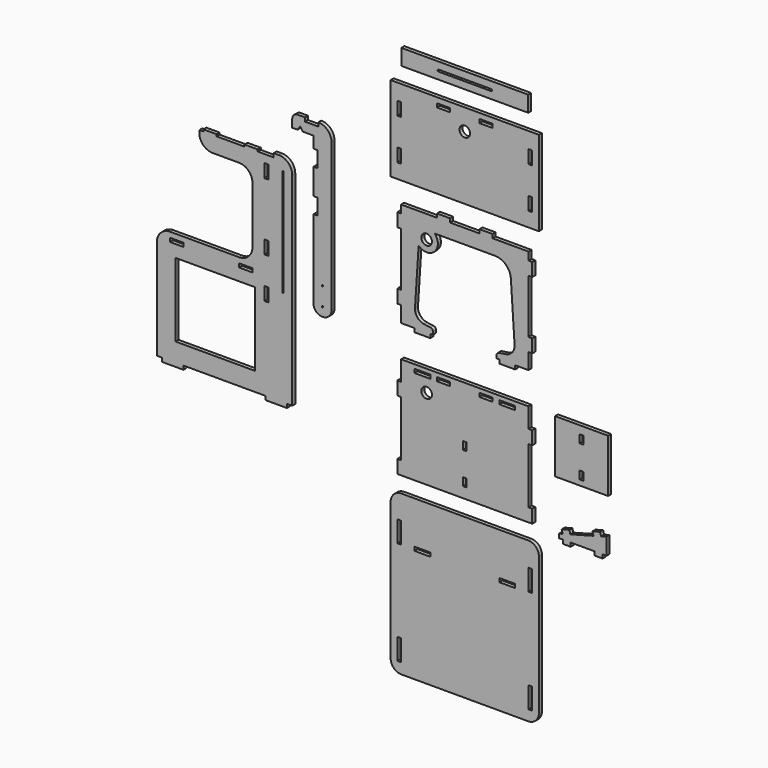
from build123d import *

# Parameters (mm, degrees)
F1_W     = 381
F1_H     = 352.425
F1_W_2   = 63.5
F1_H_2   = 18.034
F1_W_3   = 18.034
F1_H_3   = 63.5
F1_H_4   = 9.017
F1_W_4   = 101.6
F2_DEPTH = 18.034
F1_W_5   = 76.2
F1_H_5   = 38.1
F1_R     = 25.4
F1_H_6   = 101.6
F1_W_6   = 709.168
F1_H_7   = 406.4
F1_R_2   = 3.302
F1_W_7   = 607.06
F1_H_8   = 76.2
F1_W_8   = 254
F1_H_9   = 254
F1_W_9   = 38.1


# Not quite as in the source:
# - a variable given as a bare number and used for a length is read in inches; the dataset says mm whatever the document's units were
# - a feature names something its author has since deleted; it is built from what else it names


with BuildPart() as f2:
    # F1 (on Front) → F2 (new body)
    with BuildSketch(Plane.XZ):
        with BuildLine():
            Line((-279.4, -155.575), (-279.4, -635))
            Line((-279.4, -635), (-254, -635))
            Line((-254, -635), (-152.4, -635))
            Line((-152.4, -635), (241.3, -635))
            Line((241.3, -635), (279.4, -635))
            Line((279.4, -635), (342.9, -635))
            Line((342.9, -635), (368.3, -635))
            Line((368.3, -635), (368.3, 336.55))
            ThreePointArc((368.3, 336.55), (349.7012806053, 381.4512806053), (304.8, 400.05))
            Line((304.8, 400.05), (279.4, 400.05))
            Line((279.4, 400.05), (279.4, 382.016))
            Line((279.4, 382.016), (203.2, 382.016))
            Line((203.2, 382.016), (139.7, 382.016))
            Line((139.7, 382.016), (6.35, 382.016))
            Line((6.35, 382.016), (-57.15, 382.016))
            Line((-57.15, 382.016), (-76.2, 382.016))
            Line((-76.2, 382.016), (-76.2, 369.316))
            ThreePointArc((-76.2, 369.316), (-57.6012806053, 324.4147193947), (-12.7, 305.816))
            Line((-12.7, 305.816), (114.3, 305.816))
            ThreePointArc((114.3, 305.816), (159.2012806053, 287.2172806053), (177.8, 242.316))
            Line((177.8, 242.316), (177.8, -28.575))
            ThreePointArc((177.8, -28.575), (159.2012806053, -73.4762806053), (114.3, -92.075))
            Line((114.3, -92.075), (-215.9, -92.075))
            ThreePointArc((-215.9, -92.075), (-260.8012806053, -110.6737193947), (-279.4, -155.575))
        make_face()
        with Locations((0, -369.8875)):
            Rectangle(F1_W, F1_H, mode=Mode.SUBTRACT)
        with Locations((-184.15, -126.492)):
            Rectangle(F1_W_2, F1_H_2, mode=Mode.SUBTRACT)
        with Locations((244.983, -205.359)):
            Rectangle(F1_W_3, F1_H_3, mode=Mode.SUBTRACT)
        with Locations((146.05, -126.492)):
            Rectangle(F1_W_2, F1_H_2, mode=Mode.SUBTRACT)
        with Locations((244.983, -9.525)):
            Rectangle(F1_W_3, F1_H_3, mode=Mode.SUBTRACT)
        with Locations((244.983, 312.166)):
            Rectangle(F1_W_3, F1_H_3, mode=Mode.SUBTRACT)
        with BuildLine():
            Line((320.548, -171.45), (320.548, 336.55))
            ThreePointArc((320.548, 336.55), (323.85, 339.852), (327.152, 336.55))
            Line((327.152, 336.55), (327.152, -171.45))
            ThreePointArc((327.152, -171.45), (323.85, -174.752), (320.548, -171.45))
        make_face(mode=Mode.SUBTRACT)
        with Locations((-25.4, 386.5245)):
            Rectangle(F1_W_2, F1_H_4)
        with Locations((171.45, 386.5245)):
            Rectangle(F1_W_2, F1_H_4)
        with Locations((-203.2, -644.017)):
            Rectangle(F1_W_4, F1_H_2)
        Polygon((279.4, -635), (241.3, -635), (241.3, -653.034), (342.9, -653.034), (342.9, -635), align=None)
    extrude(amount=F2_DEPTH)


with BuildPart() as f2b:
    # F1 (on Front) → F2, piece 2 (new body)
    with BuildSketch(Plane.XZ):
        with BuildLine():
            Line((1028.7, -117.475), (1041.4, -117.475))
            Line((1041.4, -117.475), (1041.4, -103.0896516015))
            ThreePointArc((1041.4, -103.0896516015), (1038.2942652284, -94.7685894863), (1030.4960512242, -90.517293032))
            Line((1030.4960512242, -90.517293032), (999.0535147229, -86.0255021033))
            ThreePointArc((999.0535147229, -86.0255021033), (966.8028818472, -67.7600208894), (955.5442757756, -32.4474889188))
            Line((955.5442757756, -32.4474889188), (972.9763642782, 236.2681553483))
            Line((972.9763642782, 236.2681553483), (973.2767673279, 240.8988683598))
            ThreePointArc((973.2767673279, 240.8988683598), (977.2685807204, 260.7747670037), (986.3600521584, 278.8946750652))
            ThreePointArc((986.3600521584, 278.8946750652), (993.3552042783, 292.0453587546), (1006.5205471316, 299.0128821478))
            ThreePointArc((1006.5205471316, 299.0128821478), (1026.930915356, 308.8035329746), (1049.3169330941, 312.166))
            Line((1049.3169330941, 312.166), (1338.2830669059, 312.166))
            ThreePointArc((1338.2830669059, 312.166), (1390.3913936445, 291.5642219546), (1414.3232326721, 240.8988683598))
            Line((1414.3232326721, 240.8988683598), (1432.0557242244, -32.4474889188))
            ThreePointArc((1432.0557242244, -32.4474889188), (1420.7971181528, -67.7600208894), (1388.5464852771, -86.0255021033))
            Line((1388.5464852771, -86.0255021033), (1357.1039487758, -90.517293032))
            ThreePointArc((1357.1039487758, -90.517293032), (1349.3057347716, -94.7685894863), (1346.2, -103.0896516015))
            Line((1346.2, -103.0896516015), (1346.2, -117.475))
            Line((1346.2, -117.475), (1358.9, -117.475))
            Line((1358.9, -117.475), (1435.1, -117.475))
            Line((1435.1, -117.475), (1498.6, -117.475))
            Line((1498.6, -117.475), (1498.6, -41.275))
            Line((1498.6, -41.275), (1498.6, 22.225))
            Line((1498.6, 22.225), (1498.6, 280.416))
            Line((1498.6, 280.416), (1498.6, 343.916))
            Line((1498.6, 343.916), (1498.6, 382.016))
            Line((1498.6, 382.016), (1327.15, 382.016))
            Line((1327.15, 382.016), (1263.65, 382.016))
            Line((1263.65, 382.016), (1123.95, 382.016))
            Line((1123.95, 382.016), (1060.45, 382.016))
            Line((1060.45, 382.016), (889, 382.016))
            Line((889, 382.016), (889, 343.916))
            Line((889, 343.916), (889, 280.416))
            Line((889, 280.416), (889, 22.225))
            Line((889, 22.225), (889, -41.275))
            Line((889, -41.275), (889, -117.475))
            Line((889, -117.475), (952.5, -117.475))
            Line((952.5, -117.475), (1028.7, -117.475))
        make_face()
        with Locations((1092.2, 391.033)):
            Rectangle(F1_W_2, F1_H_2)
        with Locations((879.983, 312.166)):
            Rectangle(F1_W_3, F1_H_3)
        with Locations((879.983, -9.525)):
            Rectangle(F1_W_3, F1_H_3)
        with Locations((1507.617, -9.525)):
            Rectangle(F1_W_3, F1_H_3)
        with Locations((1397, -126.492)):
            Rectangle(F1_W_5, F1_H_2)
        with Locations((990.6, -126.492)):
            Rectangle(F1_W_5, F1_H_2)
        with Locations((1507.617, 312.166)):
            Rectangle(F1_W_3, F1_H_3)
        with Locations((1295.4, 391.033)):
            Rectangle(F1_W_2, F1_H_2)
        with BuildLine():
            Line((973.2767673279, 240.8988683598), (972.9763642782, 236.2681553483))
            ThreePointArc((972.9763642782, 236.2681553483), (1049.2460697839, 235.8954166111), (1049.3169330941, 312.166))
            ThreePointArc((1049.3169330941, 312.166), (1026.930915356, 308.8035329746), (1006.5205471316, 299.0128821478))
            ThreePointArc((1006.5205471316, 299.0128821478), (1027.4808222479, 293.6424922575), (1036.696850211, 274.066))
            ThreePointArc((1036.696850211, 274.066), (1008.8714296841, 248.7820656687), (986.3600521584, 278.8946750652))
            ThreePointArc((986.3600521584, 278.8946750652), (977.2685807204, 260.7747670037), (973.2767673279, 240.8988683598))
        make_face()
    extrude(amount=F2_DEPTH)


with BuildPart() as f2c:
    # F1 (on Front) → F2, piece 3 (new body)
    with BuildSketch(Plane.XZ):
        Polygon((1498.6, -365.125), (1498.6, -269.875), (889, -269.875), (889, -365.125), (889, -428.625), (889, -695.325), (889, -758.825), (1498.6, -758.825), (1498.6, -695.325), (1498.6, -428.625), align=None)
        with Locations((1193.8, -688.975)):
            Rectangle(F1_W_3, F1_H_5, mode=Mode.SUBTRACT)
        with Locations((1011.296850211, -371.475)):
            Circle(F1_R, mode=Mode.SUBTRACT)
        with Locations((990.6, -297.942)):
            Rectangle(F1_W_5, F1_H_2, mode=Mode.SUBTRACT)
        with Locations((1193.8, -536.575)):
            Rectangle(F1_W_3, F1_H_5, mode=Mode.SUBTRACT)
        with Locations((1092.2, -297.942)):
            Rectangle(F1_W_2, F1_H_2, mode=Mode.SUBTRACT)
        with Locations((1295.4, -297.942)):
            Rectangle(F1_W_2, F1_H_2, mode=Mode.SUBTRACT)
        with Locations((1397, -297.942)):
            Rectangle(F1_W_5, F1_H_2, mode=Mode.SUBTRACT)
        with Locations((1507.617, -727.075)):
            Rectangle(F1_W_3, F1_H_3)
        with Locations((1507.617, -396.875)):
            Rectangle(F1_W_3, F1_H_3)
        with Locations((879.983, -396.875)):
            Rectangle(F1_W_3, F1_H_3)
        with Locations((879.983, -727.075)):
            Rectangle(F1_W_3, F1_H_3)
    extrude(amount=F2_DEPTH)


with BuildPart() as f2d:
    # F1 (on Front) → F2, piece 4 (new body)
    with BuildSketch(Plane.XZ):
        with BuildLine():
            Line((1497.584, -835.025), (890.016, -835.025))
            ThreePointArc((890.016, -835.025), (854.0949755157, -849.9039755157), (839.216, -885.825))
            Line((839.216, -885.825), (839.216, -1546.225))
            ThreePointArc((839.216, -1546.225), (854.0949755157, -1582.1460244843), (890.016, -1597.025))
            Line((890.016, -1597.025), (1497.584, -1597.025))
            ThreePointArc((1497.584, -1597.025), (1533.5050244843, -1582.1460244843), (1548.384, -1546.225))
            Line((1548.384, -1546.225), (1548.384, -885.825))
            ThreePointArc((1548.384, -885.825), (1533.5050244843, -849.9039755157), (1497.584, -835.025))
        make_face()
        with Locations((879.983, -1495.425)):
            Rectangle(F1_W_3, F1_H_6, mode=Mode.SUBTRACT)
        with Locations((879.983, -1000.125)):
            Rectangle(F1_W_3, F1_H_6, mode=Mode.SUBTRACT)
        with Locations((990.6, -1047.242)):
            Rectangle(F1_W_5, F1_H_2, mode=Mode.SUBTRACT)
        with Locations((1507.617, -1495.425)):
            Rectangle(F1_W_3, F1_H_6, mode=Mode.SUBTRACT)
        with Locations((1397, -1047.242)):
            Rectangle(F1_W_5, F1_H_2, mode=Mode.SUBTRACT)
        with Locations((1507.617, -1000.125)):
            Rectangle(F1_W_3, F1_H_6, mode=Mode.SUBTRACT)
    extrude(amount=F2_DEPTH)


with BuildPart() as f2e:
    # F1 (on Front) → F2, piece 5 (new body)
    with BuildSketch(Plane.XZ):
        with Locations((1193.8, 686.816)):
            Rectangle(F1_W_6, F1_H_7)
        with Locations((879.983, 585.216)):
            Rectangle(F1_W_3, F1_H_3, mode=Mode.SUBTRACT)
        with Locations((879.983, 782.066)):
            Rectangle(F1_W_3, F1_H_3, mode=Mode.SUBTRACT)
        with Locations((1193.8, 788.416)):
            Circle(F1_R, mode=Mode.SUBTRACT)
        with Locations((1092.2, 855.599)):
            Rectangle(F1_W_2, F1_H_2, mode=Mode.SUBTRACT)
        with Locations((1295.4, 855.599)):
            Rectangle(F1_W_2, F1_H_2, mode=Mode.SUBTRACT)
        with Locations((1507.617, 585.216)):
            Rectangle(F1_W_3, F1_H_3, mode=Mode.SUBTRACT)
        with Locations((1507.617, 782.066)):
            Rectangle(F1_W_3, F1_H_3, mode=Mode.SUBTRACT)
    extrude(amount=F2_DEPTH)


with BuildPart() as f2f:
    # F1 (on Front) → F2, piece 6 (new body)
    with BuildSketch(Plane.XZ):
        with BuildLine():
            ThreePointArc((469.9, -171.45), (482.1751548005, -201.0848451995), (511.81, -213.36))
            Line((511.81, -213.36), (514.35, -213.36))
            ThreePointArc((514.35, -213.36), (543.9848451995, -201.0848451995), (556.26, -171.45))
            Line((556.26, -171.45), (556.26, 535.94))
            ThreePointArc((556.26, 535.94), (537.6612806053, 580.8412806053), (492.76, 599.44))
            Line((492.76, 599.44), (492.76, 581.406))
            Line((492.76, 581.406), (429.26, 581.406))
            Line((429.26, 581.406), (429.26, 599.44))
            Line((429.26, 599.44), (393.7, 599.44))
            ThreePointArc((393.7, 599.44), (375.7394877579, 592.0005122421), (368.3, 574.04))
            Line((368.3, 574.04), (368.3, 535.94))
            Line((368.3, 535.94), (393.7, 535.94))
            Line((393.7, 535.94), (406.4, 554.99))
            Line((406.4, 554.99), (419.1, 535.94))
            Line((419.1, 535.94), (469.9, 535.94))
            Line((469.9, 535.94), (469.9, 481.076))
            Line((469.9, 481.076), (487.934, 481.076))
            Line((487.934, 481.076), (487.934, 404.876))
            Line((487.934, 404.876), (469.9, 404.876))
            Line((469.9, 404.876), (469.9, 281.076))
            Line((469.9, 281.076), (487.934, 281.076))
            Line((487.934, 281.076), (487.934, 204.876))
            Line((487.934, 204.876), (469.9, 204.876))
            Line((469.9, 204.876), (469.9, -171.45))
        make_face()
        with Locations((513.08, -171.45)):
            Circle(F1_R_2, mode=Mode.SUBTRACT)
        with Locations((513.08, -82.55)):
            Circle(F1_R_2, mode=Mode.SUBTRACT)
    extrude(amount=F2_DEPTH)


with BuildPart() as f2g:
    # F1 (on Front) → F2, piece 7 (new body)
    with BuildSketch(Plane.XZ):
        with Locations((1193.8, 1004.316)):
            Rectangle(F1_W_7, F1_H_8)
        with BuildLine():
            Line((1319.2, 999.871), (1068.4, 999.871))
            ThreePointArc((1068.4, 999.871), (1063.955, 1004.316), (1068.4, 1008.761))
            Line((1068.4, 1008.761), (1319.2, 1008.761))
            ThreePointArc((1319.2, 1008.761), (1323.645, 1004.316), (1319.2, 999.871))
        make_face(mode=Mode.SUBTRACT)
    extrude(amount=F2_DEPTH)


with BuildPart() as f2h:
    # F1 (on Front) → F2, piece 8 (new body)
    with BuildSketch(Plane.XZ):
        with Locations((1752.6, -396.875)):
            Rectangle(F1_W_8, F1_H_9)
        with Locations((1752.6, -479.425)):
            Rectangle(F1_W_3, F1_H_5, mode=Mode.SUBTRACT)
        with Locations((1752.6, -327.025)):
            Rectangle(F1_W_3, F1_H_5, mode=Mode.SUBTRACT)
    extrude(amount=F2_DEPTH)


with BuildPart() as f2i:
    # F1 (on Front) → F2, piece 9 (new body)
    with BuildSketch(Plane.XZ):
        Polygon((1662.0348869908, -753.8944971908), (1643.634, -758.825), (1643.634, -777.875), (1662.684, -777.875), (1700.784, -777.875), (1815.084, -777.875), (1853.184, -777.875), (1872.234, -777.875), (1872.234, -697.5718146102), (1846.0437568989, -704.5894690988), (1809.2419829173, -714.4504747172), (1698.8366609724, -744.0334915724), align=None)
        Polygon((1657.3673443314, -736.4749908395), (1662.0348869908, -753.8944971908), (1698.8366609724, -744.0334915724), (1694.169118313, -726.6139852211), align=None)
        with Locations((1681.734, -786.892)):
            Rectangle(F1_W_9, F1_H_2)
        with Locations((1834.134, -786.892)):
            Rectangle(F1_W_9, F1_H_2)
        Polygon((1804.5744402579, -697.0309683659), (1809.2419829173, -714.4504747172), (1846.0437568989, -704.5894690988), (1841.3762142395, -687.1699627475), align=None)
    extrude(amount=F2_DEPTH)


solid = Compound([f2.part, f2b.part, f2c.part, f2d.part, f2e.part, f2f.part, f2g.part, f2h.part, f2i.part])
